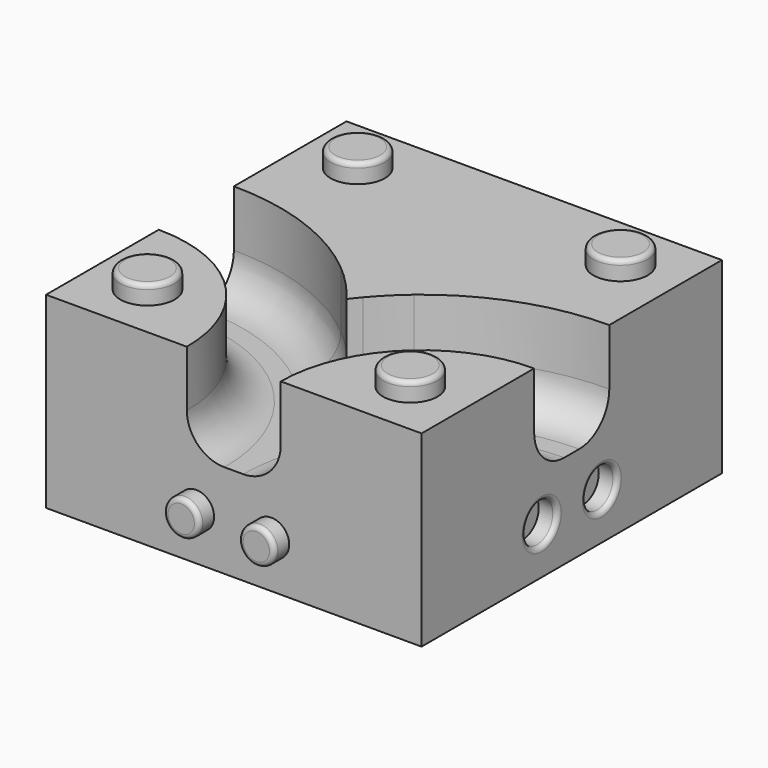
from build123d import *

# Parameters (mm, degrees)
F0_R      = 3.81
F0_R_2    = 3.937
F0_R_3    = 2.667
F0_R_4    = 3.683
F0_R_5    = 2.413
F1_DEPTH  = 12.7
F2_DEPTH  = 15.24
F3_DEPTH  = 12.7
F4_START  = -10.16
F4_DEPTH  = 2.54
F7_START  = -22.86
F6_R      = 2.413
F7_DEPTH  = 5.08
F8_START  = 22.86
F8_DEPTH  = 5.08
F9_START  = 22.86
F5_R      = 2.667
F5_R_2    = 2.413
F9_DEPTH  = 5.08
F10_START = -22.86
F10_DEPTH = 5.08
F11_START = -22.86
F6_R_2    = 2.667
F11_DEPTH = 5.08
F12_R     = 5.08
F13_R     = 0.635


# Not quite as in the source:
# - a feature names something its author has since deleted; it is built from what else it names


with BuildPart() as f1:
    # F0 (on Top) → F1 (new body)
    with BuildSketch(Plane.XY):
        with BuildLine():
            Line((25.4, 17.78), (25.4, 25.4))
            Line((25.4, 25.4), (-25.4, 25.4))
            Line((-25.4, 25.4), (-25.4, 6.35))
            ThreePointArc((-25.4, 6.35), (-14.520375766, 4.427776929), (-4.9581099388, -1.1061400612))
            ThreePointArc((-4.9581099388, -1.1061400612), (-0.5564177886, 5.0494355372), (5.08, 0))
            ThreePointArc((5.08, 0), (5.0494355372, -0.5564177886), (4.9581099388, -1.1061400612))
            ThreePointArc((4.9581099388, -1.1061400612), (14.520375766, 4.427776929), (25.4, 6.35))
            Line((25.4, 6.35), (25.4, 17.78))
        make_face()
        with Locations((-17.78, 17.78)):
            Circle(F0_R, mode=Mode.SUBTRACT)
        with Locations((17.78, 17.78)):
            Circle(F0_R_2, mode=Mode.SUBTRACT)
        with BuildLine():
            ThreePointArc((5.08, 0), (-0.5564177886, 5.0494355372), (-4.9581099388, -1.1061400612))
            ThreePointArc((-4.9581099388, -1.1061400612), (-2.9493596973, -2.9493596973), (-1.1061400612, -4.9581099388))
            ThreePointArc((-1.1061400612, -4.9581099388), (0, -5.08), (1.1061400612, -4.9581099388))
            ThreePointArc((1.1061400612, -4.9581099388), (2.9493596973, -2.9493596973), (4.9581099388, -1.1061400612))
            ThreePointArc((4.9581099388, -1.1061400612), (5.0494355372, -0.5564177886), (5.08, 0))
        make_face()
        Circle(F0_R_3, mode=Mode.SUBTRACT)
        with Locations((17.78, 17.78)):
            Circle(F0_R_2)
        with Locations((17.78, 17.78)):
            Circle(F0_R_4, mode=Mode.SUBTRACT)
        with Locations((-17.78, 17.78)):
            Circle(F0_R)
        with Locations((-17.78, 17.78)):
            Circle(F0_R_4, mode=Mode.SUBTRACT)
        with Locations((-17.78, 17.78)):
            Circle(F0_R_4)
        with Locations((17.78, 17.78)):
            Circle(F0_R_4)
        Circle(F0_R_3)
        Circle(F0_R_5, mode=Mode.SUBTRACT)
        Circle(F0_R_5)
        with BuildLine():
            ThreePointArc((1.1061400612, -4.9581099388), (0, -5.08), (-1.1061400612, -4.9581099388))
            ThreePointArc((-1.1061400612, -4.9581099388), (-0.5433254761, -5.6463109367), (0, -6.35))
            ThreePointArc((0, -6.35), (0.5433254761, -5.6463109367), (1.1061400612, -4.9581099388))
        make_face()
    extrude(amount=F1_DEPTH)

    # F0 (on Top) → F2, piece 2 (join)
    with BuildSketch(Plane.XY):
        with Locations((-17.78, 17.78)):
            Circle(F0_R_4)
        with Locations((17.78, 17.78)):
            Circle(F0_R_4)
    extrude(amount=F2_DEPTH)



with BuildPart() as f1b:
    # F0 (on Top) → F1, piece 2 (new body)
    with BuildSketch(Plane.XY):
        with BuildLine():
            ThreePointArc((-6.35, -25.4), (-11.9296158184, -11.9296158184), (-25.4, -6.35))
            Line((-25.4, -6.35), (-25.4, -25.4))
            Line((-25.4, -25.4), (-6.35, -25.4))
        make_face()
        with Locations((-17.78, -17.78)):
            Circle(F0_R, mode=Mode.SUBTRACT)
        with Locations((-17.78, -17.78)):
            Circle(F0_R)
        with Locations((-17.78, -17.78)):
            Circle(F0_R_4, mode=Mode.SUBTRACT)
        with Locations((-17.78, -17.78)):
            Circle(F0_R_4)
    extrude(amount=F1_DEPTH)

    # F0 (on Top) → F2 (join)
    with BuildSketch(Plane.XY):
        with Locations((-17.78, -17.78)):
            Circle(F0_R_4)
    extrude(amount=F2_DEPTH)


with BuildPart() as f1c:
    # F0 (on Top) → F1, piece 3 (new body)
    with BuildSketch(Plane.XY):
        with BuildLine():
            Line((25.4, -25.4), (25.4, -6.35))
            ThreePointArc((25.4, -6.35), (11.9296158184, -11.9296158184), (6.35, -25.4))
            Line((6.35, -25.4), (25.4, -25.4))
        make_face()
        with Locations((17.78, -17.78)):
            Circle(F0_R, mode=Mode.SUBTRACT)
        with Locations((17.78, -17.78)):
            Circle(F0_R)
        with Locations((17.78, -17.78)):
            Circle(F0_R_4, mode=Mode.SUBTRACT)
        with Locations((17.78, -17.78)):
            Circle(F0_R_4)
    extrude(amount=F1_DEPTH)

    # F0 (on Top) → F2, piece 3 (join)
    with BuildSketch(Plane.XY):
        with Locations((17.78, -17.78)):
            Circle(F0_R_4)
    extrude(amount=F2_DEPTH)


with BuildPart() as f1_1:
    add(f1.part)

    add(f1b.part)  # F3 merges F1b

    add(f1c.part)  # F3 merges F1c
    # F0 (on Top) → F3 (join)
    with BuildSketch(Plane.XY):
        with BuildLine():
            Line((25.4, 17.78), (25.4, 25.4))
            Line((25.4, 25.4), (-25.4, 25.4))
            Line((-25.4, 25.4), (-25.4, 6.35))
            ThreePointArc((-25.4, 6.35), (-14.520375766, 4.427776929), (-4.9581099388, -1.1061400612))
            ThreePointArc((-4.9581099388, -1.1061400612), (-0.5564177886, 5.0494355372), (5.08, 0))
            ThreePointArc((5.08, 0), (5.0494355372, -0.5564177886), (4.9581099388, -1.1061400612))
            ThreePointArc((4.9581099388, -1.1061400612), (14.520375766, 4.427776929), (25.4, 6.35))
            Line((25.4, 6.35), (25.4, 17.78))
        make_face()
        with Locations((-17.78, 17.78)):
            Circle(F0_R, mode=Mode.SUBTRACT)
        with Locations((17.78, 17.78)):
            Circle(F0_R_2, mode=Mode.SUBTRACT)
        with BuildLine():
            ThreePointArc((-4.9581099388, -1.1061400612), (-14.520375766, 4.427776929), (-25.4, 6.35))
            Line((-25.4, 6.35), (-25.4, -6.35))
            ThreePointArc((-25.4, -6.35), (-11.9296158184, -11.9296158184), (-6.35, -25.4))
            Line((-6.35, -25.4), (6.35, -25.4))
            ThreePointArc((6.35, -25.4), (11.9296158184, -11.9296158184), (25.4, -6.35))
            Line((25.4, -6.35), (25.4, 6.35))
            ThreePointArc((25.4, 6.35), (14.520375766, 4.427776929), (4.9581099388, -1.1061400612))
            ThreePointArc((4.9581099388, -1.1061400612), (3.5921024484, -3.5921024484), (1.1061400612, -4.9581099388))
            ThreePointArc((1.1061400612, -4.9581099388), (0.5433254761, -5.6463109367), (0, -6.35))
            ThreePointArc((0, -6.35), (-0.5433254761, -5.6463109367), (-1.1061400612, -4.9581099388))
            ThreePointArc((-1.1061400612, -4.9581099388), (-3.5921024484, -3.5921024484), (-4.9581099388, -1.1061400612))
        make_face()
        with BuildLine():
            ThreePointArc((-6.35, -25.4), (-11.9296158184, -11.9296158184), (-25.4, -6.35))
            Line((-25.4, -6.35), (-25.4, -25.4))
            Line((-25.4, -25.4), (-6.35, -25.4))
        make_face()
        with Locations((-17.78, -17.78)):
            Circle(F0_R, mode=Mode.SUBTRACT)
        with BuildLine():
            Line((25.4, -25.4), (25.4, -6.35))
            ThreePointArc((25.4, -6.35), (11.9296158184, -11.9296158184), (6.35, -25.4))
            Line((6.35, -25.4), (25.4, -25.4))
        make_face()
        with Locations((17.78, -17.78)):
            Circle(F0_R, mode=Mode.SUBTRACT)
        with BuildLine():
            ThreePointArc((5.08, 0), (-0.5564177886, 5.0494355372), (-4.9581099388, -1.1061400612))
            ThreePointArc((-4.9581099388, -1.1061400612), (-2.9493596973, -2.9493596973), (-1.1061400612, -4.9581099388))
            ThreePointArc((-1.1061400612, -4.9581099388), (0, -5.08), (1.1061400612, -4.9581099388))
            ThreePointArc((1.1061400612, -4.9581099388), (2.9493596973, -2.9493596973), (4.9581099388, -1.1061400612))
            ThreePointArc((4.9581099388, -1.1061400612), (5.0494355372, -0.5564177886), (5.08, 0))
        make_face()
        Circle(F0_R_3, mode=Mode.SUBTRACT)
        with Locations((17.78, 17.78)):
            Circle(F0_R_2)
        with Locations((17.78, 17.78)):
            Circle(F0_R_4, mode=Mode.SUBTRACT)
        with Locations((17.78, -17.78)):
            Circle(F0_R)
        with Locations((17.78, -17.78)):
            Circle(F0_R_4, mode=Mode.SUBTRACT)
        with Locations((-17.78, -17.78)):
            Circle(F0_R)
        with Locations((-17.78, -17.78)):
            Circle(F0_R_4, mode=Mode.SUBTRACT)
        with Locations((-17.78, 17.78)):
            Circle(F0_R)
        with Locations((-17.78, 17.78)):
            Circle(F0_R_4, mode=Mode.SUBTRACT)
        with Locations((17.78, -17.78)):
            Circle(F0_R_4)
        with Locations((-17.78, -17.78)):
            Circle(F0_R_4)
        with Locations((-17.78, 17.78)):
            Circle(F0_R_4)
        with Locations((17.78, 17.78)):
            Circle(F0_R_4)
        Circle(F0_R_3)
        Circle(F0_R_5, mode=Mode.SUBTRACT)
        Circle(F0_R_5)
        with BuildLine():
            ThreePointArc((-1.1061400612, -4.9581099388), (-2.9493596973, -2.9493596973), (-4.9581099388, -1.1061400612))
            ThreePointArc((-4.9581099388, -1.1061400612), (-3.5921024484, -3.5921024484), (-1.1061400612, -4.9581099388))
        make_face()
        with BuildLine():
            ThreePointArc((1.1061400612, -4.9581099388), (3.5921024484, -3.5921024484), (4.9581099388, -1.1061400612))
            ThreePointArc((4.9581099388, -1.1061400612), (2.9493596973, -2.9493596973), (1.1061400612, -4.9581099388))
        make_face()
        with BuildLine():
            ThreePointArc((1.1061400612, -4.9581099388), (0, -5.08), (-1.1061400612, -4.9581099388))
            ThreePointArc((-1.1061400612, -4.9581099388), (-0.5433254761, -5.6463109367), (0, -6.35))
            ThreePointArc((0, -6.35), (0.5433254761, -5.6463109367), (1.1061400612, -4.9581099388))
        make_face()
    extrude(amount=-F3_DEPTH)

    # F0 (on Top) → F4 (cut)
    with BuildSketch(Plane.XY.offset(F4_START)):
        with Locations((17.78, 17.78)):
            Circle(F0_R_2)
        with Locations((17.78, 17.78)):
            Circle(F0_R_4, mode=Mode.SUBTRACT)
        with Locations((-17.78, -17.78)):
            Circle(F0_R)
        with Locations((-17.78, -17.78)):
            Circle(F0_R_4, mode=Mode.SUBTRACT)
        with Locations((17.78, -17.78)):
            Circle(F0_R)
        with Locations((17.78, -17.78)):
            Circle(F0_R_4, mode=Mode.SUBTRACT)
        with Locations((-17.78, 17.78)):
            Circle(F0_R)
        with Locations((-17.78, 17.78)):
            Circle(F0_R_4, mode=Mode.SUBTRACT)
        with Locations((17.78, -17.78)):
            Circle(F0_R_4)
        with Locations((-17.78, -17.78)):
            Circle(F0_R_4)
        with Locations((17.78, 17.78)):
            Circle(F0_R_4)
        with Locations((-17.78, 17.78)):
            Circle(F0_R_4)
    extrude(amount=-F4_DEPTH, mode=Mode.SUBTRACT)

    # F6 (on Front) → F7 (join)
    with BuildSketch(Plane.XZ.offset(F7_START)):
        with Locations((-5.08, -6.35)):
            Circle(F6_R)
    extrude(amount=-F7_DEPTH)

    # F6 (on Front) → F8 (join)
    with BuildSketch(Plane.XZ.offset(F8_START)):
        with Locations((-5.08, -6.35)):
            Circle(F6_R)
        with Locations((5.08, -6.35)):
            Circle(F6_R)
    extrude(amount=F8_DEPTH)

    # F5 (on Right) → F9 (cut)
    with BuildSketch(Plane.YZ.offset(F9_START)):
        with Locations((-5.08, -6.35)):
            Circle(F5_R)
        with Locations((-5.08, -6.35)):
            Circle(F5_R_2, mode=Mode.SUBTRACT)
        with Locations((5.08, -6.35)):
            Circle(F5_R)
        with Locations((5.08, -6.35)):
            Circle(F5_R_2, mode=Mode.SUBTRACT)
        with Locations((-5.08, -6.35)):
            Circle(F5_R_2)
        with Locations((5.08, -6.35)):
            Circle(F5_R_2)
    extrude(amount=F9_DEPTH, mode=Mode.SUBTRACT)

    # F5 (on Right) → F10 (cut)
    with BuildSketch(Plane.YZ.offset(F10_START)):
        with Locations((-5.08, -6.35)):
            Circle(F5_R)
        with Locations((-5.08, -6.35)):
            Circle(F5_R_2, mode=Mode.SUBTRACT)
        with Locations((5.08, -6.35)):
            Circle(F5_R)
        with Locations((5.08, -6.35)):
            Circle(F5_R_2, mode=Mode.SUBTRACT)
        with Locations((-5.08, -6.35)):
            Circle(F5_R_2)
        with Locations((5.08, -6.35)):
            Circle(F5_R_2)
    extrude(amount=-F10_DEPTH, mode=Mode.SUBTRACT)

    # F6 (on Front) → F11 (cut)
    with BuildSketch(Plane.XZ.offset(F11_START)):
        with Locations((5.08, -6.35)):
            Circle(F6_R_2)
        with Locations((5.08, -6.35)):
            Circle(F6_R, mode=Mode.SUBTRACT)
        with Locations((5.08, -6.35)):
            Circle(F6_R)
    extrude(amount=-F11_DEPTH, mode=Mode.SUBTRACT)

    # F12
    f12_edges = [f1_1.edges().sort_by_distance(p)[0] for p in [
        (11.929616, -11.929616, 0),
        (-11.929616, -11.929616, 0),
        (-11.200968, 2.998063, 0),
        (11.200968, 2.998063, 0),
    ]]
    fillet(f12_edges, radius=F12_R)

    # F13
    f13_edges = [f1_1.edges().sort_by_distance(p)[0] for p in [
        (14.097, -17.78, 15.24),
        (-21.463, -17.78, 15.24),
        (-21.463, 17.78, 15.24),
        (14.097, 17.78, 15.24),
        (-7.493, 27.94, -6.35),
        (-25.4, -7.747, -6.35),
        (-25.4, 2.413, -6.35),
        (2.667, -27.94, -6.35),
        (-7.493, -27.94, -6.35),
        (25.4, -7.747, -6.35),
        (25.4, 2.413, -6.35),
        (13.97, -17.78, -12.7),
        (-21.59, -17.78, -12.7),
        (13.843, 17.78, -12.7),
        (-21.59, 17.78, -12.7),
        (2.413, 25.4, -6.35),
    ]]
    fillet(f13_edges, radius=F13_R)


solid = f1_1.part
